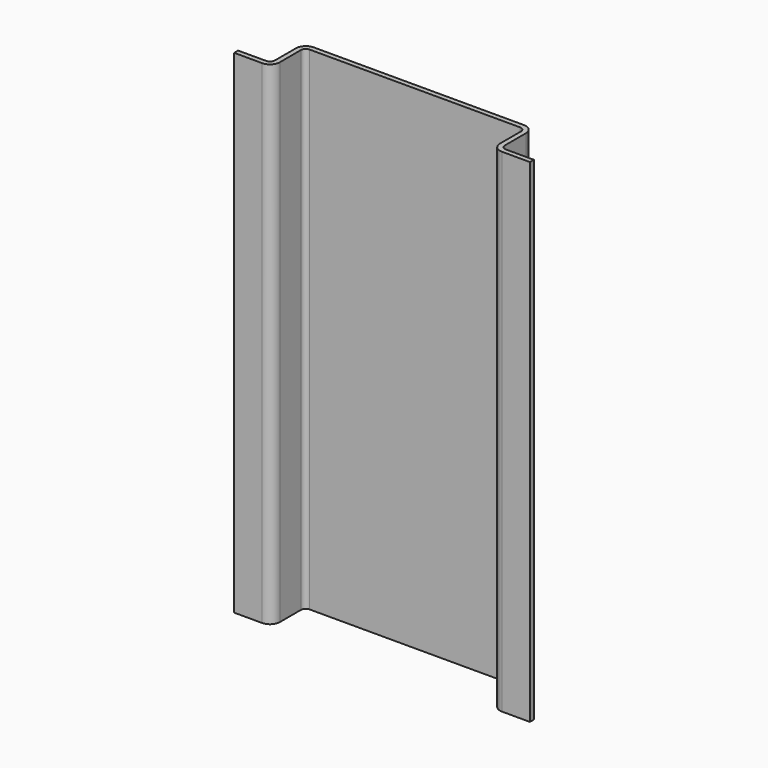
from build123d import *

# Parameters (mm, degrees)
F0_W        = 140
F0_H        = 25
F1_DEPTH    = 150
F2_T        = 3
F2_T3_DEPTH = 306
F3_R        = 3
F4_R        = 6


# Not quite as in the source:
# - a shell that OpenCascade refuses in one call is made with other operations: the cavity is built on its own and cut out


with BuildPart() as f1:
    # F0 (on Top) → F1 (new body, symmetric)
    with BuildSketch(Plane.XY):
        with Locations((40, 15.5)):
            Rectangle(F0_W, F0_H)
        Polygon((110, 3), (-30, 3), (-50, 3), (-50, 0), (130, 0), (130, 3), align=None)
    extrude(amount=F1_DEPTH, both=True)

    # F2: shell of thickness 3, made by hand


with BuildPart() as f2_core1:
    # F2_t2: copy of F1
    add(f1.part)

    # the walls: a layer under each face that stays
    f2_faces = [f2_core1.faces().sort_by_distance(p)[0] for p in [
        (-30, 15.5, 0),
        (40, 28, 0),
        (110, 15.5, 0),
        (120, 3, 0),
        (130, 1.5, 0),
        (-50, 1.5, 0),
        (-40, 3, 0),
    ]]
    thicken(f2_faces, amount=-F2_T, mode=Mode.SUBTRACT)

    # F2_s4 → F2_t3 (cut)
    with BuildSketch(Plane.XY.offset(-153)):
        Polygon((-30.03, 3.03), (-27, 3), (-27, 0), (-30, 0), align=None)
        Polygon((110.03, 3.03), (107, 3), (107, 0), (110, 0), align=None)
    extrude(amount=F2_T3_DEPTH, mode=Mode.SUBTRACT)


with BuildPart() as f1_1:
    add(f1.part)

    # what is left inside the walls is the cavity
    f2_cavity = [f2_core1.part.solids().sort_by_distance(p)[0] for p in [
        (40, 0.03, -50),
    ]]
    add(f2_cavity, mode=Mode.SUBTRACT)

    # F3
    f3_edges = [f1_1.edges().sort_by_distance(p)[0] for p in [
        (-30, 3, 0),
        (110, 3, 0),
        (-27, 25, 0),
        (107, 25, 0),
    ]]
    fillet(f3_edges, radius=F3_R)

    # F4
    f4_edges = [f1_1.edges().sort_by_distance(p)[0] for p in [
        (-27, 0, 0),
        (107, 0, 0),
        (-30, 28, 0),
        (110, 28, 0),
    ]]
    fillet(f4_edges, radius=F4_R)


solid = f1_1.part
